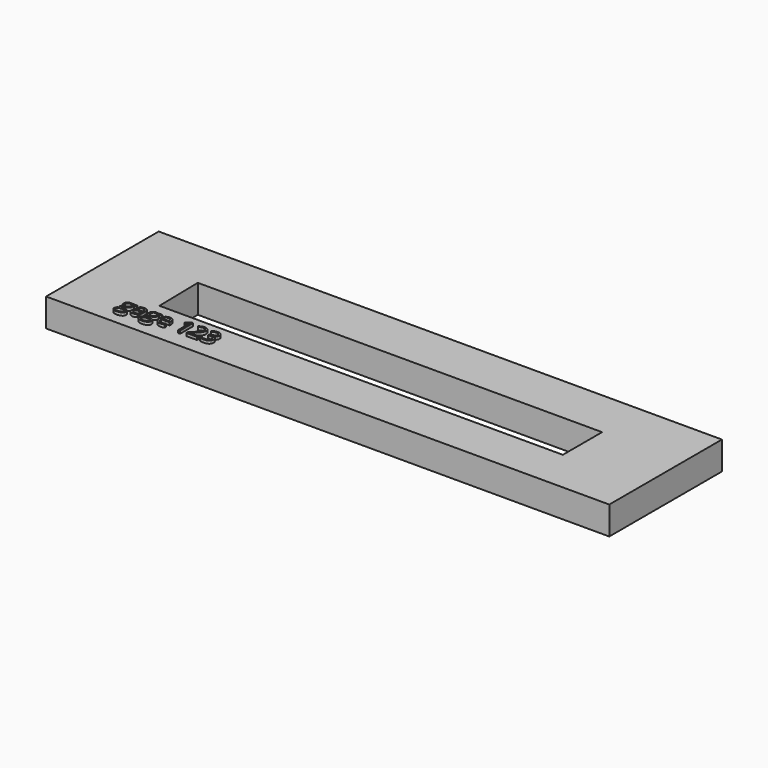
from build123d import *

# Parameters (mm, degrees)
F0_W         = 200
F0_H         = 50
F1_DEPTH     = 10
F3_DEPTH     = 25
F4_TEXT_SIZE = 8.1274296261
F5_DEPTH     = 1


# Not quite as in the source:
# - Text() gives the source's letters only with a copy of the font that has no kerning and outlines rounded to 1/6400 em; it was checked with that copy


with BuildPart() as f1:
    # F0 (on Top) → F1 (new body)
    with BuildSketch(Plane.XY):
        with Locations((4.2615045931, -18.1541059365)):
            Rectangle(F0_W, F0_H)
    extrude(amount=F1_DEPTH)

    # F2 (on face) → F3 (cut)
    with BuildSketch(Plane.XY.offset(10)):
        Polygon((-68.0257230997, -10.4527715594), (-67.7232220769, -27.8751235455), (75.5496025085, -27.8751235455), (75.5496025085, -10.4527715594), align=None)
    extrude(amount=-F3_DEPTH, mode=Mode.SUBTRACT)

    # F4 (on face) → F5 (join)
    with BuildSketch(Plane.XY.offset(10)):
        with Locations((-75.6617039442, -37.4467037618)):
            Text('gage 123', F4_TEXT_SIZE, font='Open Sans', text_align=(TextAlign.LEFT, TextAlign.BOTTOM))
    extrude(amount=F5_DEPTH)


solid = f1.part
